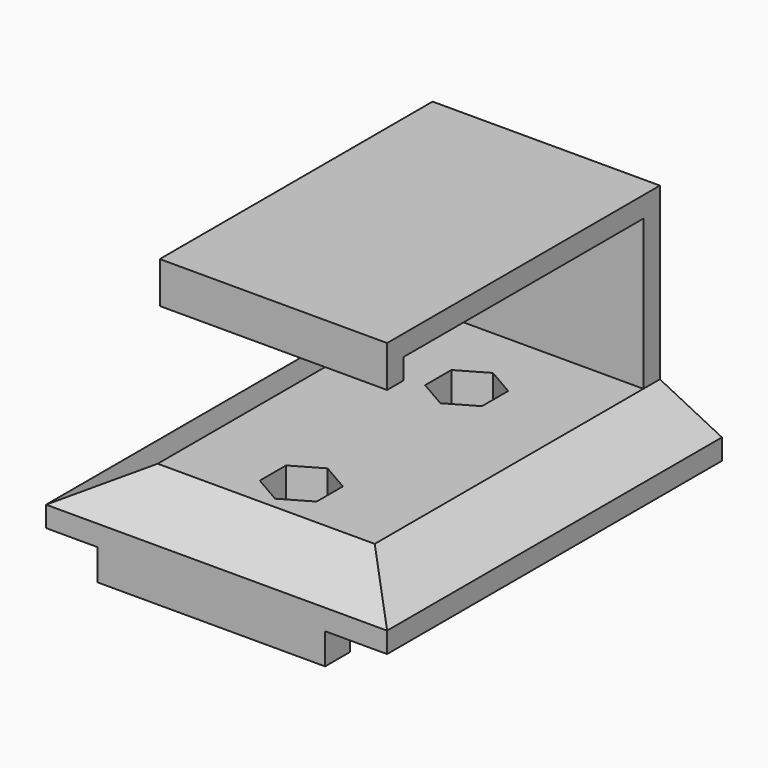
from build123d import *

# Parameters (mm, degrees)
F0_W          = 2
F0_H          = 14.5
F0_W_2        = 3
F0_H_2        = 3
F0_W_3        = 29
F0_H_3        = 2
F1_DEPTH      = 22
F2_DEPTH      = 28
F2_DEPTH_BACK = 5
F3_R          = 1.75
F4_DEPTH      = 5
F5_START      = -1
F5_DEPTH      = 4
F6_SIZE2      = 3
F6_SIZE       = 6


# Not quite as in the source:
# - a feature names something its author has since deleted; it is built from what else it names


with BuildPart() as f1:
    # F0 (on Right) → F1 (new body)
    with BuildSketch(Plane.YZ):
        Polygon((-20.25, 5), (-20.25, 0), (-17.25, 0), (17.25, 0), (20.25, 0), (20.25, 5), (18.25, 5), align=None)
        with Locations((19.25, 12.25)):
            Rectangle(F0_W, F0_H)
        with Locations((-18.75, -1.5)):
            Rectangle(F0_W_2, F0_H_2)
        with Locations((18.75, -1.5)):
            Rectangle(F0_W_2, F0_H_2)
        with Locations((3.75, 20.5)):
            Rectangle(F0_W_3, F0_H_3)
        with Locations((19.25, 20.5)):
            Rectangle(F0_W, F0_H_3)
        Polygon((-10.75, 17.5), (-10.75, 19.5), (-10.75, 21.5), (-12.75, 21.5), (-12.75, 17.5), align=None)
    extrude(amount=F1_DEPTH)

    # F0 (on Right) → F2 (join, two sides)
    with BuildSketch(Plane.YZ) as f2_sk:
        Polygon((-20.25, 5), (-20.25, 0), (-17.25, 0), (17.25, 0), (20.25, 0), (20.25, 5), (18.25, 5), align=None)
    extrude(amount=F2_DEPTH)
    extrude(f2_sk.sketch, amount=-F2_DEPTH_BACK)

    # F3 (on face) → F4 (cut, through all)
    with BuildSketch(Plane(origin=(0, 0, 0), x_dir=(1, 0, 0), z_dir=(0, 0, -1))):
        with Locations((11.5, 10)):
            Circle(F3_R)
        with Locations((11.5, -10)):
            Circle(F3_R)
    extrude(amount=-F4_DEPTH, mode=Mode.SUBTRACT)

    # F3 (on face) → F5 (cut)
    with BuildSketch(Plane(origin=(0, 0, 0), x_dir=(1, 0, 0), z_dir=(0, 0, -1)).offset(F5_START)):
        Polygon((8.75, -8.4122867597), (8.75, -11.5877132403), (11.5, -13.1754264805), (14.25, -11.5877132403), (14.25, -8.4122867597), (11.5, -6.8245735195), align=None)
        with Locations((11.5, -10)):
            Circle(F3_R, mode=Mode.SUBTRACT)
        Polygon((8.75, 11.5877132403), (8.75, 8.4122867597), (11.5, 6.8245735195), (14.25, 8.4122867597), (14.25, 11.5877132403), (11.5, 13.1754264805), align=None)
        with Locations((11.5, 10)):
            Circle(F3_R, mode=Mode.SUBTRACT)
    extrude(amount=-F5_DEPTH, mode=Mode.SUBTRACT)

    # F6
    f6_edges = [f1.edges().sort_by_distance(p)[0] for p in [
        (28, 0, 5),
        (11.5, -20.25, 5),
        (-5, 0, 5),
    ]]
    f6_side = f1.faces().sort_by_distance((11.51774, -0.683006, 5))[0]
    chamfer(f6_edges, length=F6_SIZE, length2=F6_SIZE2, reference=f6_side)


solid = f1.part
